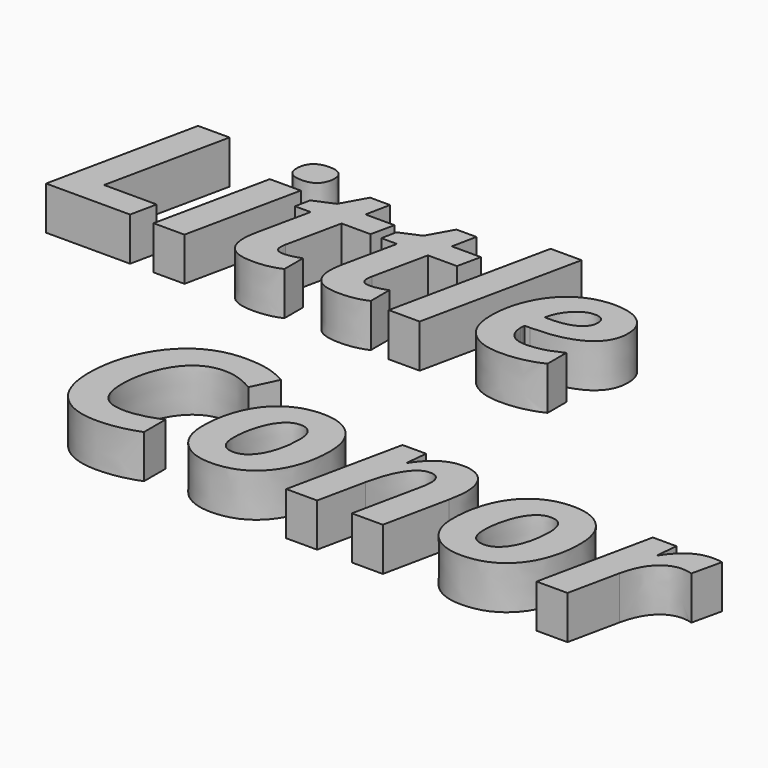
from build123d import *

# Parameters (mm, degrees)
F0_TEXT_SIZE = 30.8680555556
F1_DEPTH     = 6.35


# Not quite as in the source:
# - Text() gives the source's letters only with a copy of the font that has no kerning and outlines rounded to 1/6400 em; it was checked with that copy


with BuildPart() as f1:
    # F0 (on Top) → F1 (new body)
    with BuildSketch(Plane.XY):
        with Locations((0, 0)):
            Text('Little', F0_TEXT_SIZE, font='Open Sans', font_style=FontStyle.BOLDITALIC, text_align=(TextAlign.LEFT, TextAlign.BOTTOM))
        with Locations((32.0834852431, -41.9805555556)):
            Text('Conor', F0_TEXT_SIZE, font='Open Sans', font_style=FontStyle.BOLDITALIC, text_align=(TextAlign.LEFT, TextAlign.BOTTOM))
    extrude(amount=F1_DEPTH)


solid = f1.part
